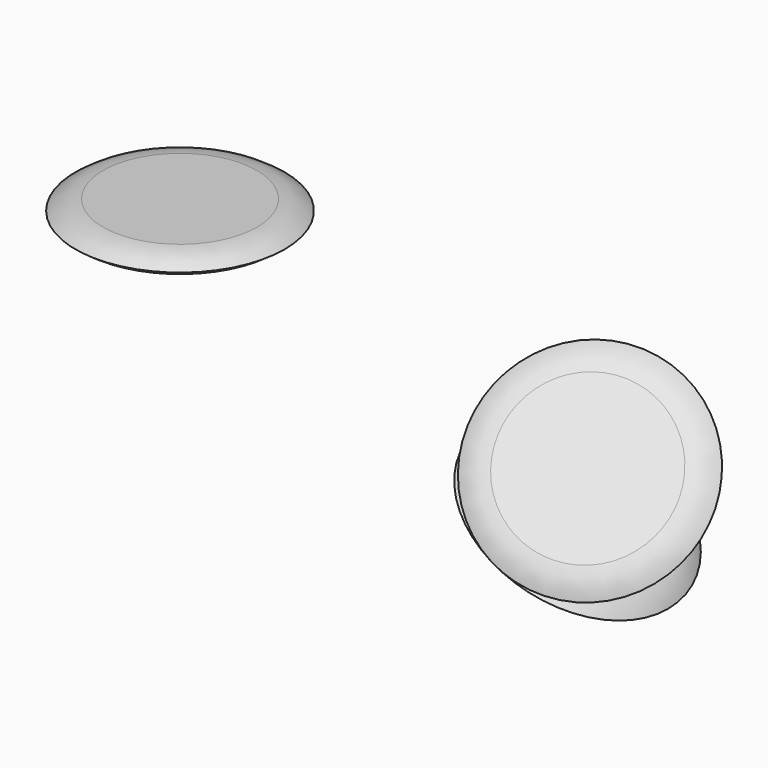
from build123d import *

# Parameters (mm, degrees)
F0_R      = 12.7
F1_DEPTH  = 1.27
F2_SIZE   = 1.26999
F8_ANGLE  = -30
F11_ANGLE = -45


# Not quite as in the source:
# - a fillet or chamfer that OpenCascade refuses, or shapes differently, is made with other operations: its cross-section is extruded or revolved along the edge and cut away or added
# - a fillet or chamfer is up to 0.001 mm smaller than in the source, because OpenCascade refuses the exact size


with BuildPart() as f1:
    # F0 (on Top) → F1 (new body, symmetric)
    with BuildSketch(Plane.XY):
        Circle(F0_R)
    extrude(amount=F1_DEPTH, both=True)

    # F2 (size 1.27 in the source; OpenCascade refuses exactly that, so slightly less here)
    f2_edges = [f1.edges().sort_by_distance(p)[0] for p in [
        (-12.7, 0, -1.27),
        (-12.7, 0, 1.27),
    ]]
    chamfer(f2_edges, length=F2_SIZE)

    # F3: fillet of radius 5.08 on 1 edges, made by hand

    # F3_s1 → F3_t2 (revolve, cut)
    with BuildSketch(Plane.XZ):
        with BuildLine():
            ThreePointArc((12.7, 1e-05), (11.135951327, 0.9419075538), (9.3399071739, 1.27))
            Line((9.3399071739, 1.27), (11.43001, 1.27))
            Line((11.43001, 1.27), (12.7, 1e-05))
        make_face()
    revolve(axis=Axis((0, 0, 1.27), (0, 0, 1)), mode=Mode.SUBTRACT)

    # F4: fillet of radius 5.08 on 1 edges, made by hand

    # F4_s1 → F4_t2 (revolve, cut)
    with BuildSketch(Plane.XZ):
        with BuildLine():
            ThreePointArc((12.7, -1e-05), (11.135951327, -0.9419075538), (9.3399071739, -1.27))
            Line((9.3399071739, -1.27), (11.43001, -1.27))
            Line((11.43001, -1.27), (12.7, -1e-05))
        make_face()
    revolve(axis=Axis((0, 0, -1.27), (0, 0, 1)), mode=Mode.SUBTRACT)


with BuildPart() as f5_1:
    # F5: copy of F1
    add(f1.part.moved(Location((38.1, 12.7, -25.4))))


with BuildPart() as f5_1_1:
    # F8: moved
    add(f5_1.part.rotate(Axis((38.1, 17.4700720236, -25.4), (0, -1, 0)), F8_ANGLE))


with BuildPart() as f11_1:
    # F11: copy of F5_1
    add(f5_1_1.part.rotate(Axis((33.3806926878, 0, -22.6753066529), (-0.8660254038, 0, 0.5)), F11_ANGLE))


solid = Compound([f1.part, f5_1_1.part, f11_1.part])
